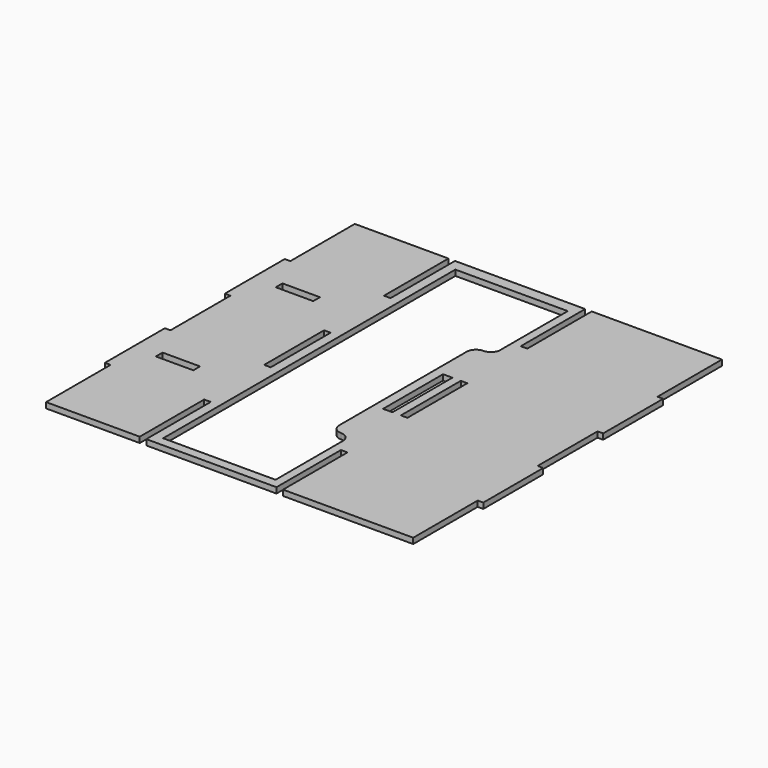
from build123d import *

# Parameters (mm, degrees)
F0_W     = 3.5
F0_H     = 40
F0_W_2   = 5
F1_DEPTH = 3
F2_R     = 5
F3_R     = 4.99999
F4_R     = 4.99999


# Not quite as in the source:
# - a fillet or chamfer is up to 0.001 mm smaller than in the source, because OpenCascade refuses the exact size


with BuildPart() as f1:
    # F0 (on Top) → F1 (new body)
    with BuildSketch(Plane.XY):
        Polygon((129.5, -200), (199, -200), (199, -157), (202, -157), (202, -117), (199, -117), (199, -77), (202, -77), (202, -37), (199, -37), (199, 6), (129.5, 6), (129.5, -37), (126, -37), (126, 6), (56.5, 6), (56.5, -37), (53, -37), (53, 6), (3, 6), (3, -37), (0, -37), (0, -77), (3, -77), (3, -117), (0, -117), (0, -157), (3, -157), (3, -200), (53, -200), (53, -157), (56.5, -157), (56.5, -200), (126, -200), (126, -157), (129.5, -157), align=None)
        Polygon((33, -134.75), (33, -137), (33, -139.25), (13, -139.25), (13, -134.75), align=None, mode=Mode.SUBTRACT)
        with Locations((54.75, -97)):
            Rectangle(F0_W, F0_H, mode=Mode.SUBTRACT)
        Polygon((61.5, -195), (61.5, -97), (61.5, 0), (121.5, 0), (121.5, -50), (111.5, -50), (111.5, -145), (121.5, -145), (121.5, -195), align=None, mode=Mode.SUBTRACT)
        with Locations((119, -97)):
            Rectangle(F0_W_2, F0_H, mode=Mode.SUBTRACT)
        with Locations((127.75, -97)):
            Rectangle(F0_W, F0_H, mode=Mode.SUBTRACT)
        Polygon((33, -54.75), (33, -57), (33, -59.25), (13, -59.25), (13, -54.75), align=None, mode=Mode.SUBTRACT)
    extrude(amount=F1_DEPTH)

    # F2
    f2_edges = [f1.edges().sort_by_distance(p)[0] for p in [
        (121.5, -50, 1.5),
    ]]
    fillet(f2_edges, radius=F2_R)

    # F3 (radius 5 in the source; OpenCascade refuses exactly that, so slightly less here)
    f3_edges = [f1.edges().sort_by_distance(p)[0] for p in [
        (111.5, -50, 1.5),
    ]]
    fillet(f3_edges, radius=F3_R)

    # F4 (radius 5 in the source; OpenCascade refuses exactly that, so slightly less here)
    f4_edges = [f1.edges().sort_by_distance(p)[0] for p in [
        (121.5, -145, 1.5),
        (111.5, -145, 1.5),
    ]]
    fillet(f4_edges, radius=F4_R)


solid = f1.part
